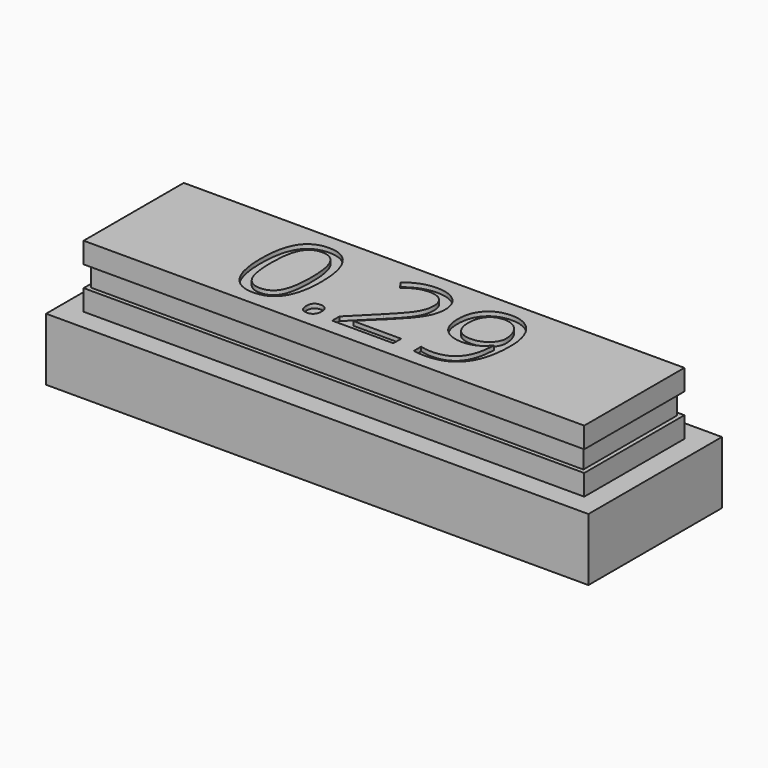
from build123d import *

# Parameters (mm, degrees)
F0_W         = 26
F0_H         = 8
F0_W_2       = 20
F0_H_2       = 2
F1_DEPTH     = 3
F2_W         = 24
F2_H         = 6
F3_DEPTH     = 3
F5_W         = 24
F5_H         = 6
F5_W_2       = 23.6
F5_H_2       = 5.6
F6_DEPTH     = 0.5
F7_W         = 19.42
F7_H         = 1.42
F8_DEPTH     = 3
F9_TEXT_SIZE = 6.25
F10_DEPTH    = 0.2


# Not quite as in the source:
# - Text() gives the source's letters only with a copy of the font that has no kerning and outlines rounded to 1/6400 em; it was checked with that copy


with BuildPart() as f1:
    # F0 (on Top) → F1 (new body)
    with BuildSketch(Plane.XY):
        Rectangle(F0_W, F0_H)
        Rectangle(F0_W_2, F0_H_2, mode=Mode.SUBTRACT)
    extrude(amount=F1_DEPTH)


with BuildPart() as f3:
    # F2 (on face) → F3 (new body)
    with BuildSketch(Plane.XY.offset(3)):
        Rectangle(F2_W, F2_H)
    extrude(amount=F3_DEPTH)

    # F5 (on mid) → F6 (cut, symmetric)
    with BuildSketch(Plane.XY.offset(4.5)):
        Rectangle(F5_W, F5_H)
        Rectangle(F5_W_2, F5_H_2, mode=Mode.SUBTRACT)
    extrude(amount=F6_DEPTH, both=True, mode=Mode.SUBTRACT)

    # F7 (on face) → F8 (join, through all)
    with BuildSketch(Plane(origin=(0, 0, 3), x_dir=(1, 0, 0), z_dir=(0, 0, -1))):
        Rectangle(F7_W, F7_H)
    extrude(amount=F8_DEPTH)

    # F9 (on face) → F10 (cut)
    with BuildSketch(Plane.XY.offset(6)):
        with Locations((-6.2265625, -2.25)):
            Text('0.29', F9_TEXT_SIZE, font='Open Sans', text_align=(TextAlign.LEFT, TextAlign.BOTTOM))
    extrude(amount=-F10_DEPTH, mode=Mode.SUBTRACT)


solid = Compound([f1.part, f3.part])
